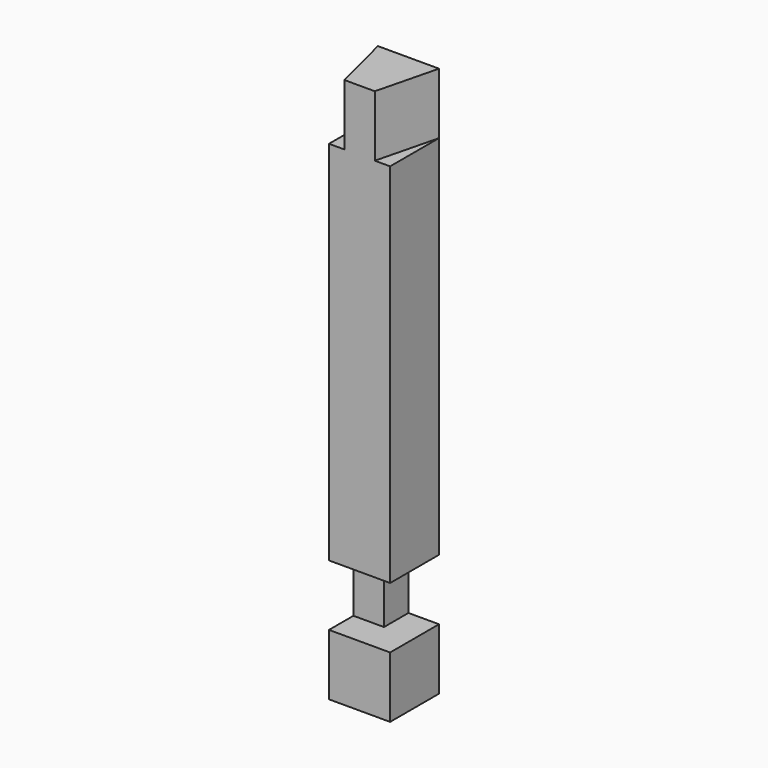
from build123d import *

# Parameters (mm, degrees)
F0_W     = 101.6
F0_H     = 101.6
F1_DEPTH = 914.4
F3_DEPTH = 101.6
F4_W     = 101.6
F4_H     = 101.6
F5_DEPTH = 50.8
F6_W     = 50.8
F6_H     = 101.6
F7_DEPTH = 50.8


with BuildPart() as f1:
    # F0 (on Top) → F1 (new body)
    with BuildSketch(Plane.XY):
        Rectangle(F0_W, F0_H)
    extrude(amount=F1_DEPTH)

    # F2 (on face) → F3 (cut)
    with BuildSketch(Plane.XY.offset(914.4)):
        Polygon((-25.4, -50.8), (-50.8, 50.8), (-50.8, -50.8), align=None)
        Polygon((50.8, -50.8), (50.8, 50.8), (25.4, -50.8), align=None)
    extrude(amount=-F3_DEPTH, mode=Mode.SUBTRACT)

    # F4 (on face) → F5 (cut)
    with BuildSketch(Plane.XZ.offset(50.8)):
        with Locations((0, 152.4)):
            Rectangle(F4_W, F4_H)
    extrude(amount=-F5_DEPTH, mode=Mode.SUBTRACT)

    # F6 (on face) → F7 (cut)
    with BuildSketch(Plane.YZ.offset(50.8)):
        with Locations((25.4, 152.4)):
            Rectangle(F6_W, F6_H)
    extrude(amount=-F7_DEPTH, mode=Mode.SUBTRACT)


solid = f1.part
